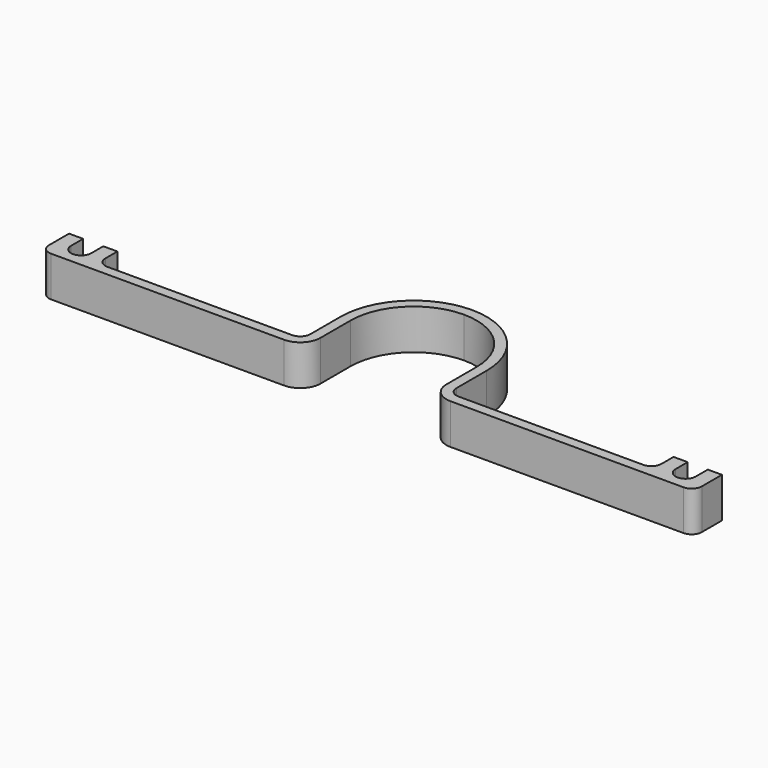
from build123d import *

# Parameters (mm, degrees)
F1_DEPTH = 4
F2_R     = 0.99999
F3_R     = 2
F4_W     = 1.4
F4_H     = 4
F5_DEPTH = 1.5
F6_R     = 1


# Not quite as in the source:
# - a fillet or chamfer is up to 0.001 mm smaller than in the source, because OpenCascade refuses the exact size


with BuildPart() as f1:
    # F0 (on Top) → F1 (new body)
    with BuildSketch(Plane.XY):
        with BuildLine():
            Line((-6.25, -5.75), (-6.25, -3.6742346142))
            ThreePointArc((-6.25, -3.6742346142), (-6.9955342898, -1.9039432765), (-7.25, 0))
            Line((-7.25, 0), (-7.25, -4.75))
            Line((-7.25, -4.75), (-27.6, -4.75))
            Line((-27.6, -4.75), (-27.6, -3.75))
            Line((-27.6, -3.75), (-29, -3.75))
            ThreePointArc((-29, -3.75), (-30, -4.75), (-31, -3.75))
            Line((-31, -3.75), (-32.4, -3.75))
            ThreePointArc((-32.4, -3.75), (-31.6928932188, -4.0428932188), (-31.4, -4.75))
            ThreePointArc((-31.4, -4.75), (-31.6928932188, -5.4571067812), (-32.4, -5.75))
            Line((-32.4, -5.75), (-6.25, -5.75))
        make_face()
        with BuildLine():
            Line((-32.4, -3.75), (-32.4, -5.75))
            ThreePointArc((-32.4, -5.75), (-31.6928932188, -5.4571067812), (-31.4, -4.75))
            ThreePointArc((-31.4, -4.75), (-31.6928932188, -4.0428932188), (-32.4, -3.75))
        make_face()
        with BuildLine():
            ThreePointArc((-6.25, 0), (-4.4194173824, 4.4194173824), (0, 6.25))
            Line((0, 6.25), (0, 7.25))
            ThreePointArc((0, 7.25), (-5.1265241636, 5.1265241636), (-7.25, 0))
            ThreePointArc((-7.25, 0), (-6.9955342898, -1.9039432765), (-6.25, -3.6742346142))
            Line((-6.25, -3.6742346142), (-6.25, 0))
        make_face()
    extrude(amount=F1_DEPTH)

    # F2 (radius 1 in the source; OpenCascade refuses exactly that, so slightly less here)
    f2_edges = [f1.edges().sort_by_distance(p)[0] for p in [
        (-27.6, -4.75, 2),
        (-7.25, -4.75, 2),
    ]]
    fillet(f2_edges, radius=F2_R)

    # F3
    f3_edges = [f1.edges().sort_by_distance(p)[0] for p in [
        (-6.25, -5.75, 2),
    ]]
    fillet(f3_edges, radius=F3_R)

    # F4 (on face) → F5 (join)
    with BuildSketch(Plane(origin=(0, -3.75, 0), x_dir=(-1, 0, 0), z_dir=(0, 1, 0))):
        with Locations((28.3, 2)):
            Rectangle(F4_W, F4_H)
        with Locations((31.7, 2)):
            Rectangle(F4_W, F4_H)
    extrude(amount=F5_DEPTH)

    # F6
    f6_edges = [f1.edges().sort_by_distance(p)[0] for p in [
        (-32.4, -5.75, 2),
    ]]
    fillet(f6_edges, radius=F6_R)

    # F7: F1 across plane


with BuildPart() as f1_1:
    add(f1.part)
    add(f1.part.mirror(Plane.YZ))


solid = f1_1.part
